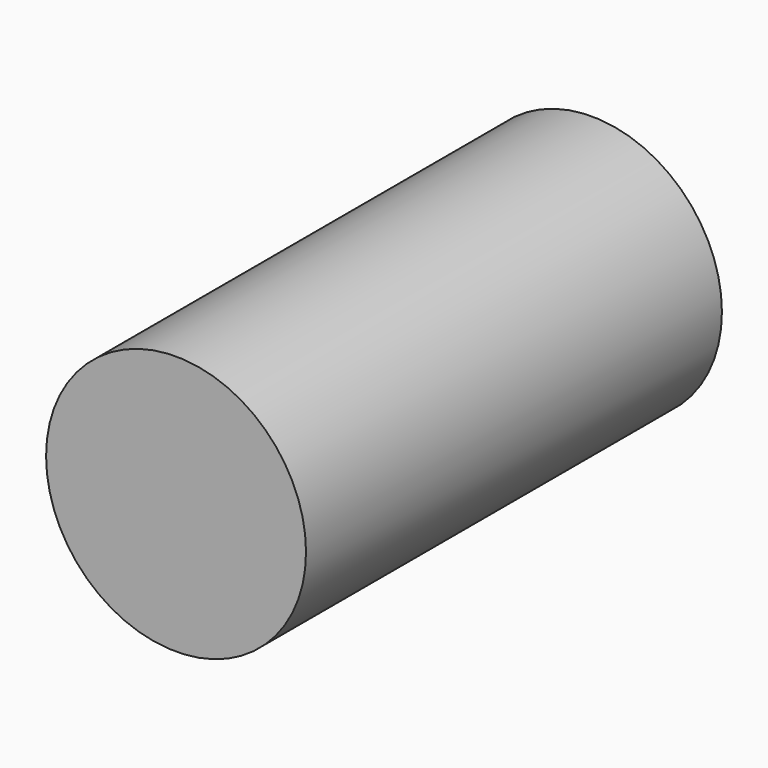
from build123d import *

# Parameters (mm, degrees)
F1_R     = 114.3
F2_DEPTH = 457.2
F3_T     = -2.54


# Not quite as in the source:
# - a variable given as a bare number and used for a length is read in inches; the dataset says mm whatever the document's units were


with BuildPart() as f2:
    # F1 (on Front) → F2 (new body)
    with BuildSketch(Plane.XZ):
        Circle(F1_R)
    extrude(amount=-F2_DEPTH)

    # F3 (hollow: no face is removed)
    offset(amount=F3_T, mode=Mode.SUBTRACT)


solid = f2.part
